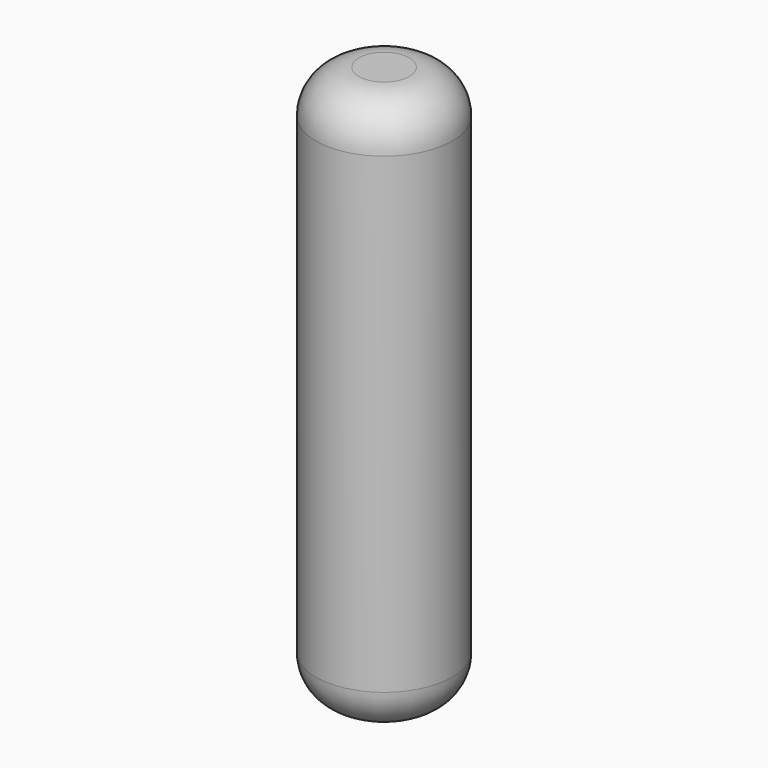
from build123d import *

# Parameters (mm, degrees)
F3_R     = 1.5875
F4_DEPTH = 13
F5_R     = 1


with BuildPart() as f4:
    # F3 (on Top) → F4 (new body)
    with BuildSketch(Plane.XY):
        Circle(F3_R)
    extrude(amount=F4_DEPTH)

    # F5
    f5_edges = [f4.edges().sort_by_distance(p)[0] for p in [
        (-1.5875, 0, 13),
        (-1.5875, 0, 0),
    ]]
    fillet(f5_edges, radius=F5_R)


solid = f4.part
